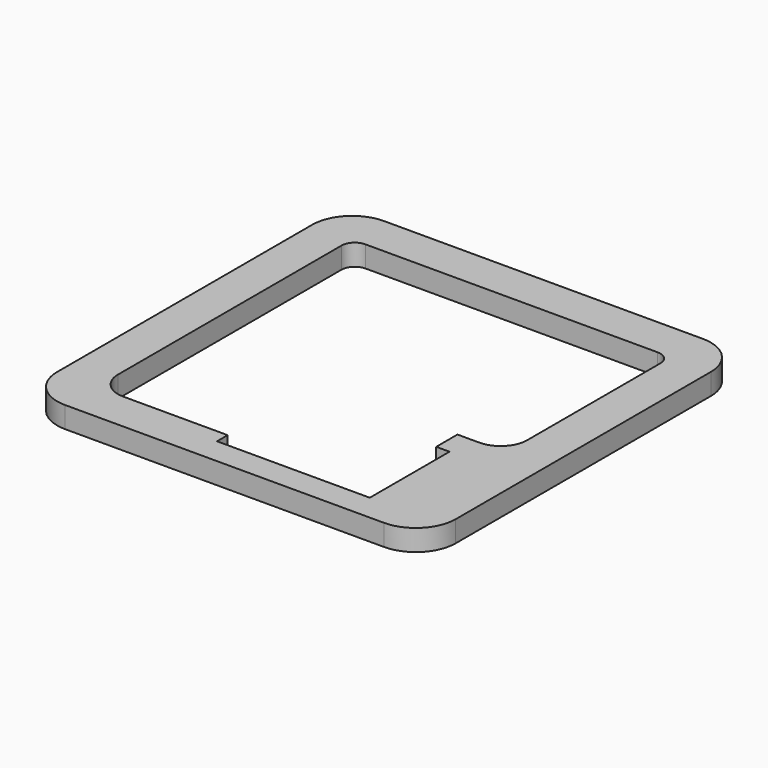
from build123d import *

# Parameters (mm, degrees)
F1_DEPTH = 1.6


# Not quite as in the source:
# - a feature names something its author has since deleted; it is built from what else it names


with BuildPart() as f1:
    # F0 (on Top) → F1 (new body)
    with BuildSketch(Plane.XY):
        with BuildLine():
            ThreePointArc((15, 12), (14.1213203436, 14.1213203436), (12, 15))
            Line((12, 15), (-12, 15))
            ThreePointArc((-12, 15), (-14.1213203436, 14.1213203436), (-15, 12))
            Line((-15, 12), (-15, -12))
            ThreePointArc((-15, -12), (-14.1213203436, -14.1213203436), (-12, -15))
            Line((-12, -15), (12, -15))
            ThreePointArc((12, -15), (14.1213203436, -14.1213203436), (15, -12))
            Line((15, -12), (15, 12))
        make_face()
        with BuildLine():
            Line((9.35, -13.025), (-2.15, -13.025))
            Line((-2.15, -13.025), (-2.15, -12.025))
            Line((-2.15, -12.025), (-10, -12.025))
            ThreePointArc((-10, -12.025), (-11.4142135624, -11.4392135624), (-12, -10.025))
            Line((-12, -10.025), (-12, 11))
            ThreePointArc((-12, 11), (-11.7071067812, 11.7071067812), (-11, 12))
            Line((-11, 12), (11, 12))
            ThreePointArc((11, 12), (11.7071067812, 11.7071067812), (12, 11))
            Line((12, 11), (12, -1.525))
            ThreePointArc((12, -1.525), (11.4142135624, -2.9392135624), (10, -3.525))
            Line((10, -3.525), (8.35, -3.525))
            Line((8.35, -3.525), (8.35, -5.525))
            Line((8.35, -5.525), (9.35, -5.525))
            Line((9.35, -5.525), (9.35, -13.025))
        make_face(mode=Mode.SUBTRACT)
    extrude(amount=F1_DEPTH)


solid = f1.part
